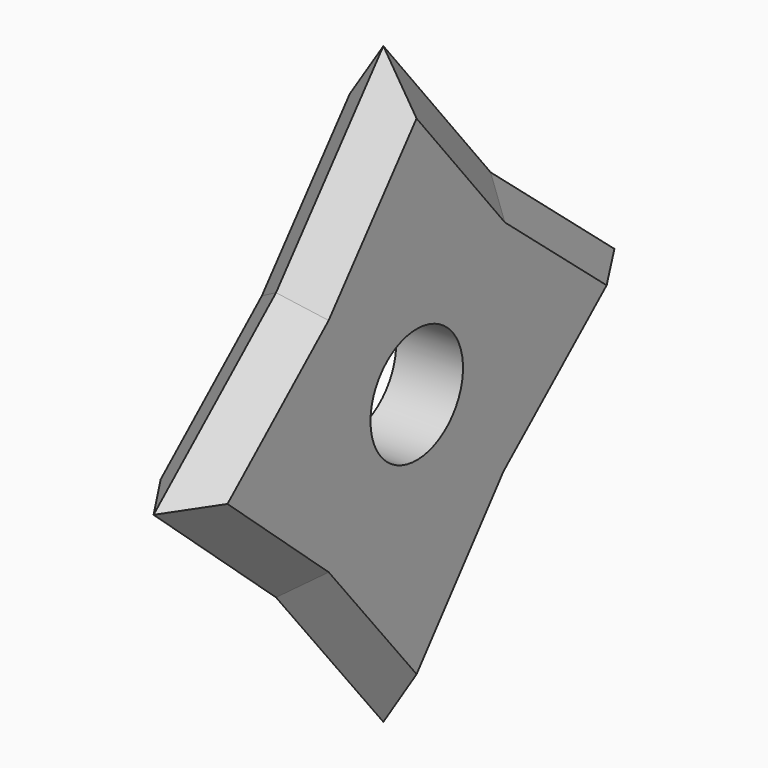
from build123d import *

# Parameters (mm, degrees)
F1_DEPTH = 12.7
F2_SIZE  = 6.34999
F4_D     = 22


# Not quite as in the source:
# - a fillet or chamfer is up to 0.001 mm smaller than in the source, because OpenCascade refuses the exact size


with BuildPart() as f1:
    # F0 (on Right) → F1 (new body)
    with BuildSketch(Plane.YZ):
        Polygon((0, 56.2922134995), (-25.5191382021, 25.3690239042), (-54.6409785748, 0), (-25.5191382021, -25.6692506373), (0, -56.8926632404), (25.2189133316, -25.6692506373), (54.9412034452, 0), (25.5191363394, 24.768576026), align=None)
    extrude(amount=F1_DEPTH)

    # F2 (size 6.35 in the source; OpenCascade refuses exactly that, so slightly less here)
    f2_edges = [f1.edges().sort_by_distance(p)[0] for p in [
        (12.7, -40.080058, 12.684512),
        (0, -40.080058, 12.684512),
        (12.7, -40.080058, -12.834625),
        (0, -40.080058, -12.834625),
        (12.7, -12.759569, -41.280957),
        (0, -12.759569, -41.280957),
        (0, 12.609457, -41.280957),
        (12.7, 12.609457, -41.280957),
        (0, 40.080058, -12.834625),
        (12.7, 40.080058, -12.834625),
        (12.7, 40.23017, 12.384288),
        (0, 40.23017, 12.384288),
        (0, 12.759568, 40.530395),
        (12.7, 12.759568, 40.530395),
        (0, -12.759569, 40.830619),
        (12.7, -12.759569, 40.830619),
    ]]
    chamfer(f2_edges, length=F2_SIZE)

    # F4 (through all)
    with Locations(Plane(origin=(0, 0, 0), x_dir=(0, 1, 0), z_dir=(-1, 0, 0))):
        with Locations((0, 0)):
            Hole(F4_D / 2)


solid = f1.part
